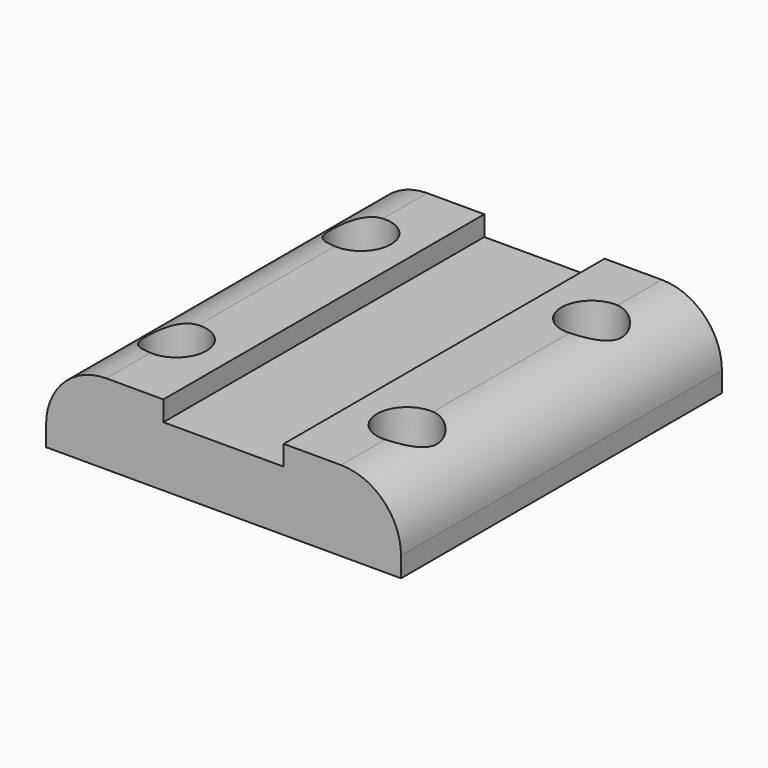
from build123d import *

# Parameters (mm, degrees)
F0_R        = 1.5
F1_DEPTH    = 4
F2_DEPTH    = 3
F3_T1_DEPTH = 35


# Not quite as in the source:
# - a fillet or chamfer that OpenCascade refuses, or shapes differently, is made with other operations: its cross-section is extruded or revolved along the edge and cut away or added


with BuildPart() as f1:
    # F0 (on Top) → F1 (new body)
    with BuildSketch(Plane.XY):
        Polygon((-8.85, -10), (-3, -10), (-3, -7.3377132403), (-5.75, -8.9254264805), (-8.5, -7.3377132403), (-8.5, -4.1622867597), (-5.75, -2.5745735195), (-3, -4.1622867597), (-3, 4.1622867597), (-5.75, 2.5745735195), (-8.5, 4.1622867597), (-8.5, 7.3377132403), (-5.75, 8.9254264805), (-3, 7.3377132403), (-3, 10), (-8.85, 10), align=None)
        Polygon((-5.75, -8.9254264805), (-3, -7.3377132403), (-3, -4.1622867597), (-5.75, -2.5745735195), (-8.5, -4.1622867597), (-8.5, -7.3377132403), align=None)
        with Locations((-5.75, -5.75)):
            Circle(F0_R, mode=Mode.SUBTRACT)
        Polygon((-3, 4.1622867597), (-3, 7.3377132403), (-5.75, 8.9254264805), (-8.5, 7.3377132403), (-8.5, 4.1622867597), (-5.75, 2.5745735195), align=None)
        with Locations((-5.75, 5.75)):
            Circle(F0_R, mode=Mode.SUBTRACT)
    extrude(amount=F1_DEPTH)



with BuildPart() as f1b:
    # F0 (on Top) → F1, piece 2 (new body)
    with BuildSketch(Plane.XY):
        Polygon((3, -10), (8.85, -10), (8.85, 10), (3, 10), (3, 7.3377132403), (5.75, 8.9254264805), (8.5, 7.3377132403), (8.5, 4.1622867597), (5.75, 2.5745735195), (3, 4.1622867597), (3, -4.1622867597), (5.75, -2.5745735195), (8.5, -4.1622867597), (8.5, -7.3377132403), (5.75, -8.9254264805), (3, -7.3377132403), align=None)
        Polygon((3, -4.1622867597), (3, -7.3377132403), (5.75, -8.9254264805), (8.5, -7.3377132403), (8.5, -4.1622867597), (5.75, -2.5745735195), align=None)
        with Locations((5.75, -5.75)):
            Circle(F0_R, mode=Mode.SUBTRACT)
        Polygon((5.75, 8.9254264805), (3, 7.3377132403), (3, 4.1622867597), (5.75, 2.5745735195), (8.5, 4.1622867597), (8.5, 7.3377132403), align=None)
        with Locations((5.75, 5.75)):
            Circle(F0_R, mode=Mode.SUBTRACT)
    extrude(amount=F1_DEPTH)


with BuildPart() as f1_1:
    add(f1.part)

    add(f1b.part)  # F2 merges F1b
    # F0 (on Top) → F2 (join)
    with BuildSketch(Plane.XY):
        Polygon((-3, -10), (0, -10), (0, 10), (-3, 10), (-3, 7.3377132403), (-3, 4.1622867597), (-3, -4.1622867597), (-3, -7.3377132403), align=None)
        Polygon((0, -10), (3, -10), (3, -7.3377132403), (3, -4.1622867597), (3, 4.1622867597), (3, 7.3377132403), (3, 10), (0, 10), align=None)
    extrude(amount=F2_DEPTH)

    # F3: fillet of radius 3 on 2 edges, made by hand

    # F3_s2 → F3_t1 (cut)
    with BuildSketch(Plane.XZ.offset(-17.5)):
        with BuildLine():
            ThreePointArc((8.85, 1), (7.9713203436, 3.1213203436), (5.85, 4))
            Line((5.85, 4), (8.85, 4))
            Line((8.85, 4), (8.85, 1))
        make_face()
        with BuildLine():
            ThreePointArc((-5.85, 4), (-7.9713203436, 3.1213203436), (-8.85, 1))
            Line((-8.85, 1), (-8.85, 4))
            Line((-8.85, 4), (-5.85, 4))
        make_face()
    extrude(amount=F3_T1_DEPTH, mode=Mode.SUBTRACT)


solid = f1_1.part
